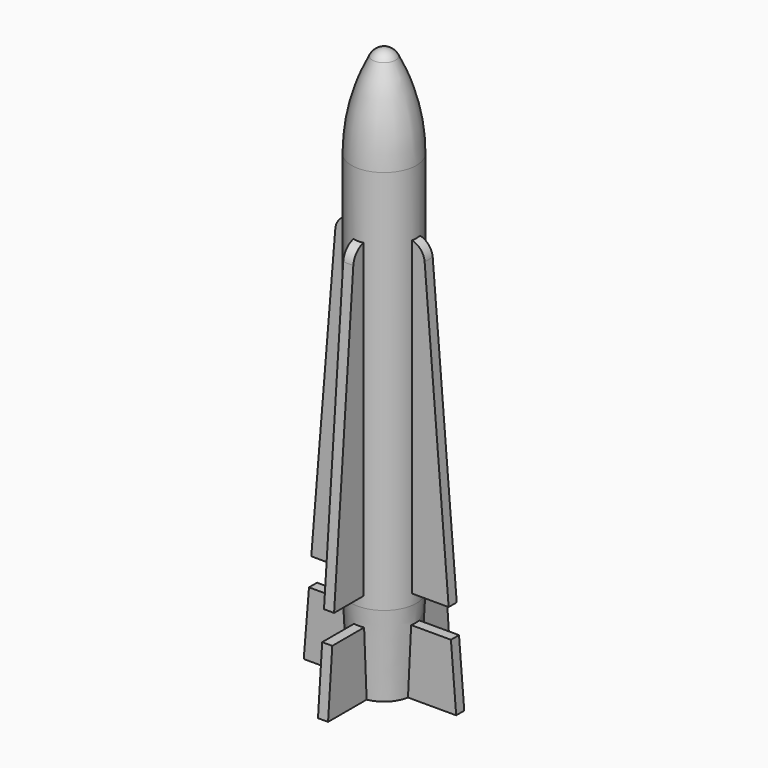
from build123d import *

# Parameters (mm, degrees)
F3_DEPTH = 0.2
F4_COUNT = 4


# Not quite as in the source:
# - a feature names something its author has since deleted; it is built from what else it names


with BuildPart() as f1:
    # F0 (on Front) → F1 (revolve)
    with BuildSketch(Plane.XZ):
        with BuildLine():
            Line((0, 22.2222222222), (0, 0))
            Line((0, 0), (1.1284722222, 0))
            Line((1.1284722222, 0), (1.2847222222, 3.2638888889))
            Line((1.2847222222, 3.2638888889), (1.2847222222, 18.5416666667))
            ThreePointArc((1.2847222222, 18.5416666667), (1.074687159, 20.2927272078), (0.4564979348, 21.9444444444))
            ThreePointArc((0.4564979348, 21.9444444444), (0.2671847948, 22.1473201826), (0, 22.2222222222))
        make_face()
    revolve(axis=Axis((0, 0, 11.1111111111), (0, 0, 1)))

    # F2 (on Front) → F3 (join, symmetric)
    with BuildSketch(Plane.XZ):
        Polygon((0, 3.2638888889), (0, 0), (3.0208333333, 0), (2.8125, 2.5694444444), (0.4, 2.5694444444), (0.4, 3.2638888889), align=None)
        with BuildLine():
            Line((0, 16.0250628992), (0, 3.2638888889))
            Line((0, 3.2638888889), (0.4, 3.2638888889))
            Line((0.4, 3.2638888889), (0.4, 3.6805555556))
            Line((0.4, 3.6805555556), (2.7224099099, 3.6805555556))
            Line((2.7224099099, 3.6805555556), (1.7708333333, 15.4166666667))
            ThreePointArc((1.7708333333, 15.4166666667), (1.5598257716, 15.8497451466), (1.1111111111, 16.0250628992))
            Line((1.1111111111, 16.0250628992), (0, 16.0250628992))
        make_face()
    extrude(amount=F3_DEPTH, both=True)

    # F4: F1 ×4 about axis
    f4_axis = Axis((0, 0, 3.2638888889), (0, 0, 1))


with BuildPart() as f1_1:
    add(f1.part)
    for i in range(1, F4_COUNT):
        add(f1.part.rotate(f4_axis, i * 360 / F4_COUNT))


solid = f1_1.part
